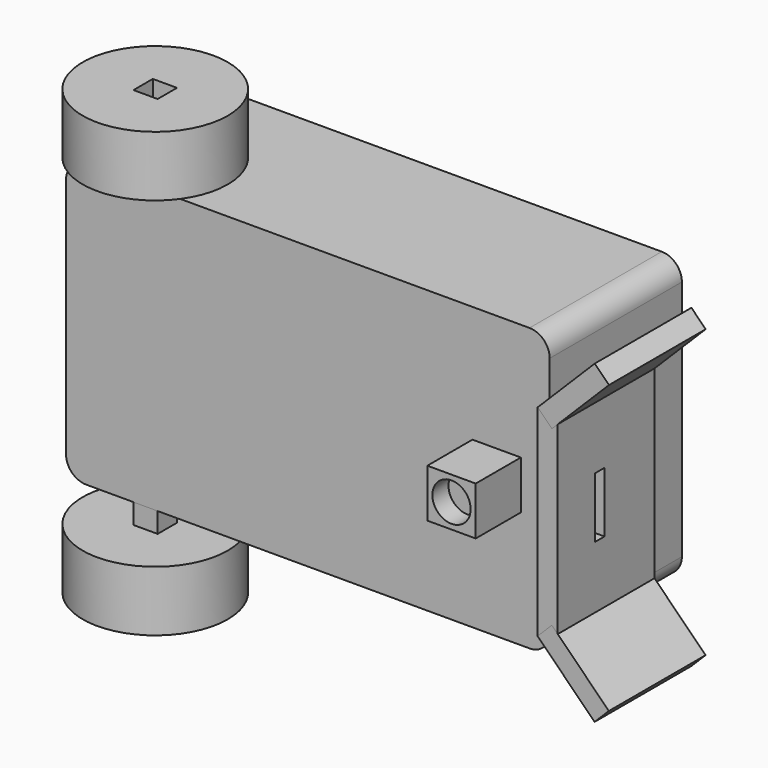
from build123d import *

# Parameters (mm, degrees)
F1_DEPTH  = 6
F2_W      = 6
F2_H      = 6
F3_DEPTH  = 5
F4_R      = 18
F5_DEPTH  = 15
F6_W      = 6
F6_H      = 6
F7_DEPTH  = 5
F8_R      = 18
F9_DEPTH  = 15
F10_W     = 12
F10_H     = 12
F11_DEPTH = 14
F12_R     = 4.7477500175
F13_DEPTH = 5
F14_W     = 3
F14_H     = 15
F15_DEPTH = 5
F16_W     = 30
F16_H     = 50
F16_W_2   = 3
F16_H_2   = 15
F17_DEPTH = 5
F18_W     = 30
F18_H     = 5
F19_DEPTH = 20
F20_ANGLE = 45
F22_ANGLE = -45
F24_W     = 5
F24_H     = 60
F25_DEPTH = 35


# Not quite as in the source:
# - a feature names something its author has since deleted; it is built from what else it names


with BuildPart() as f1:
    # F0 (on Front) → F1 (new body)
    with BuildSketch(Plane.XZ):
        with BuildLine():
            Line((55, 35), (-55, 35))
            ThreePointArc((-55, 35), (-58.5355339059, 33.5355339059), (-60, 30))
            Line((-60, 30), (-60, -30))
            ThreePointArc((-60, -30), (-58.5355339059, -33.5355339059), (-55, -35))
            Line((-55, -35), (55, -35))
            ThreePointArc((55, -35), (58.5355339059, -33.5355339059), (60, -30))
            Line((60, -30), (60, 30))
            ThreePointArc((60, 30), (58.5355339059, 33.5355339059), (55, 35))
        make_face()
    extrude(amount=F1_DEPTH)

    # F10 (on face) → F11 (join)
    with BuildSketch(Plane.XZ.offset(6)):
        with Locations((46.8423552811, 0)):
            Rectangle(F10_W, F10_H)
    extrude(amount=F11_DEPTH)

    # F12 (on face) → F13 (cut)
    with BuildSketch(Plane.XZ.offset(20)):
        with Locations((46.8423552811, 0)):
            Circle(F12_R)
    extrude(amount=-F13_DEPTH, mode=Mode.SUBTRACT)

    # F14 (on face) → F15 (join)
    with BuildSketch(Plane.YZ.offset(60)):
        with Locations((-3, 0)):
            Rectangle(F14_W, F14_H)
    extrude(amount=F15_DEPTH)

    # F24 (on face) → F25 (join)
    with BuildSketch(Plane(origin=(0, 0, 0), x_dir=(-1, 0, 0), z_dir=(0, 1, 0))):
        with BuildLine():
            Line((55, 35), (-55, 35))
            ThreePointArc((-55, 35), (-58.5355339059, 33.5355339059), (-60, 30))
            Line((-60, 30), (-55, 30))
            Line((-55, 30), (55, 30))
            Line((55, 30), (60, 30))
            ThreePointArc((60, 30), (58.5355339059, 33.5355339059), (55, 35))
        make_face()
        with Locations((-57.5, 0)):
            Rectangle(F24_W, F24_H)
        with BuildLine():
            Line((-55, -30), (-60, -30))
            ThreePointArc((-60, -30), (-58.5355339059, -33.5355339059), (-55, -35))
            Line((-55, -35), (55, -35))
            ThreePointArc((55, -35), (58.5355339059, -33.5355339059), (60, -30))
            Line((60, -30), (55, -30))
            Line((55, -30), (-55, -30))
        make_face()
        with Locations((57.5, 0)):
            Rectangle(F24_W, F24_H)
    extrude(amount=F25_DEPTH)


with BuildPart() as f3:
    # F2 (on face) → F3 (new body)
    with BuildSketch(Plane(origin=(0, 0, -35), x_dir=(1, 0, 0), z_dir=(0, 0, -1))):
        with Locations((-40.2774014771, 3)):
            Rectangle(F2_W, F2_H)
    extrude(amount=F3_DEPTH)


with BuildPart() as f5:
    # F4 (on face) → F5 (new body)
    with BuildSketch(Plane(origin=(0, 0, -40), x_dir=(1, 0, 0), z_dir=(0, 0, -1))):
        with Locations((-40.2774014771, 3)):
            Circle(F4_R)
        Polygon((-43.2774014771, 6), (-37.2774014771, 6), (-37.2774014771, 3), (-37.2774014771, 0), (-43.2774014771, 0), align=None, mode=Mode.SUBTRACT)
    extrude(amount=F5_DEPTH)


with BuildPart() as f7:
    # F6 (on face) → F7 (new body)
    with BuildSketch(Plane.XY.offset(35)):
        with Locations((-40.2774, -3)):
            Rectangle(F6_W, F6_H)
    extrude(amount=F7_DEPTH)


with BuildPart() as f9:
    # F8 (on face) → F9 (new body)
    with BuildSketch(Plane.XY.offset(40)):
        with Locations((-40.2774, -3)):
            Circle(F8_R)
        Polygon((-43.2774, 0), (-37.2774, 0), (-37.2774, -6), (-43.2774, -6), (-43.2774, -3), align=None, mode=Mode.SUBTRACT)
    extrude(amount=F9_DEPTH)


with BuildPart() as f17:
    # F16 (on face) → F17 (new body)
    with BuildSketch(Plane.YZ.offset(65)):
        with Locations((-1, 0)):
            Rectangle(F16_W, F16_H)
        with Locations((-3, 0)):
            Rectangle(F16_W_2, F16_H_2, mode=Mode.SUBTRACT)
    extrude(amount=F17_DEPTH)


with BuildPart() as f19:
    # F18 (on face) → F19 (new body)
    with BuildSketch(Plane.YZ.offset(70)):
        with Locations((-1, 22.5)):
            Rectangle(F18_W, F18_H)
    extrude(amount=F19_DEPTH)


with BuildPart() as f19b:
    # F18 (on face) → F19, piece 2 (new body)
    with BuildSketch(Plane.YZ.offset(70)):
        with Locations((-1, -22.5)):
            Rectangle(F18_W, F18_H)
    extrude(amount=F19_DEPTH)


with BuildPart() as f19_1:
    # F20: moved
    add(f19.part.rotate(Axis((70, -1, 25), (0, -1, 0)), F20_ANGLE))


with BuildPart() as f19_2:
    # F21: moved
    add(f19_1.part.moved(Location((-4.97, 0, 0))))


with BuildPart() as f19b_1:
    # F22: moved
    add(f19b.part.rotate(Axis((70, -1, -25), (0, -1, 0)), F22_ANGLE))


with BuildPart() as f19b_2:
    # F23: moved
    add(f19b_1.part.moved(Location((-5, 0, 0))))


solid = Compound([f1.part, f3.part, f5.part, f7.part, f9.part, f17.part, f19_2.part, f19b_2.part])
